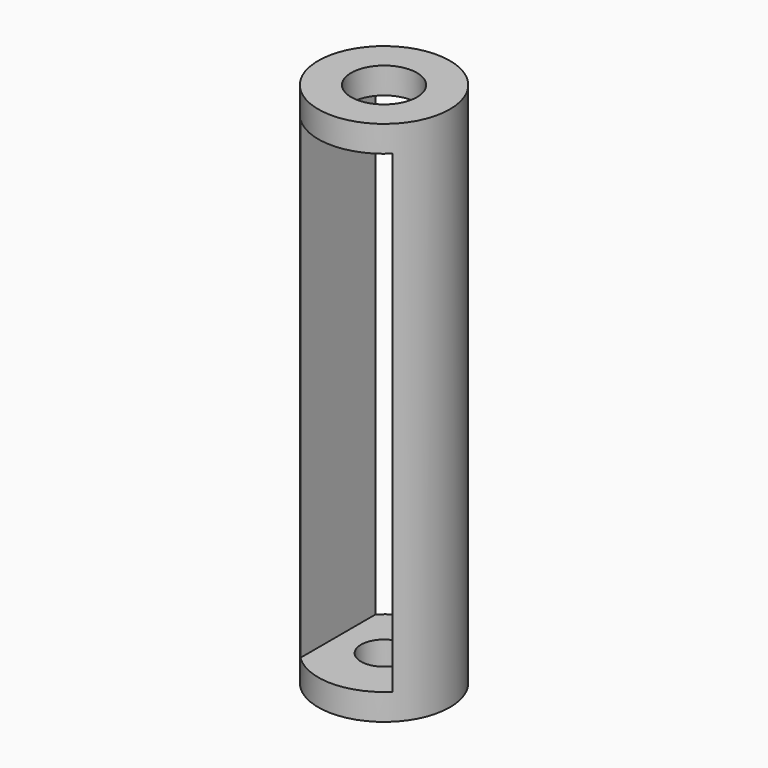
from build123d import *

# Parameters (mm, degrees)
F0_R          = 12.7
F1_DEPTH      = 101.6
F2_T          = -9.525
F3_W          = 8.89
F3_H          = 91.44
F4_DEPTH      = 12.701
F4_DEPTH_BACK = 25.4
F5_R          = 6.35
F6_DEPTH      = 25.4
F7_R          = 4.445
F8_DEPTH      = 25.4


# Not quite as in the source:
# - a length typed as a fraction of an inch, garbled in the dataset ("3 / 203.2 mm" for 3/8 in), is restored


with BuildPart() as f1:
    # F0 (on Top) → F1 (new body)
    with BuildSketch(Plane.XY):
        Circle(F0_R)
    extrude(amount=F1_DEPTH)

    # F2 (hollow: no face is removed)
    offset(amount=F2_T, mode=Mode.SUBTRACT)

    # F3 (on Front) → F4 (cut, two sides)
    with BuildSketch(Plane.XZ) as f4_sk:
        with Locations((-4.445, 50.8)):
            Rectangle(F3_W, F3_H)
        with Locations((4.445, 50.8)):
            Rectangle(F3_W, F3_H)
    extrude(amount=-F4_DEPTH, mode=Mode.SUBTRACT)
    extrude(f4_sk.sketch, amount=F4_DEPTH_BACK, mode=Mode.SUBTRACT)

    # F5 (on face) → F6 (cut)
    with BuildSketch(Plane.XY.offset(101.6)):
        Circle(F5_R)
    extrude(amount=-F6_DEPTH, mode=Mode.SUBTRACT)

    # F7 (on face) → F8 (cut)
    with BuildSketch(Plane.XY.offset(5.08)):
        Circle(F7_R)
    extrude(amount=-F8_DEPTH, mode=Mode.SUBTRACT)


solid = f1.part
